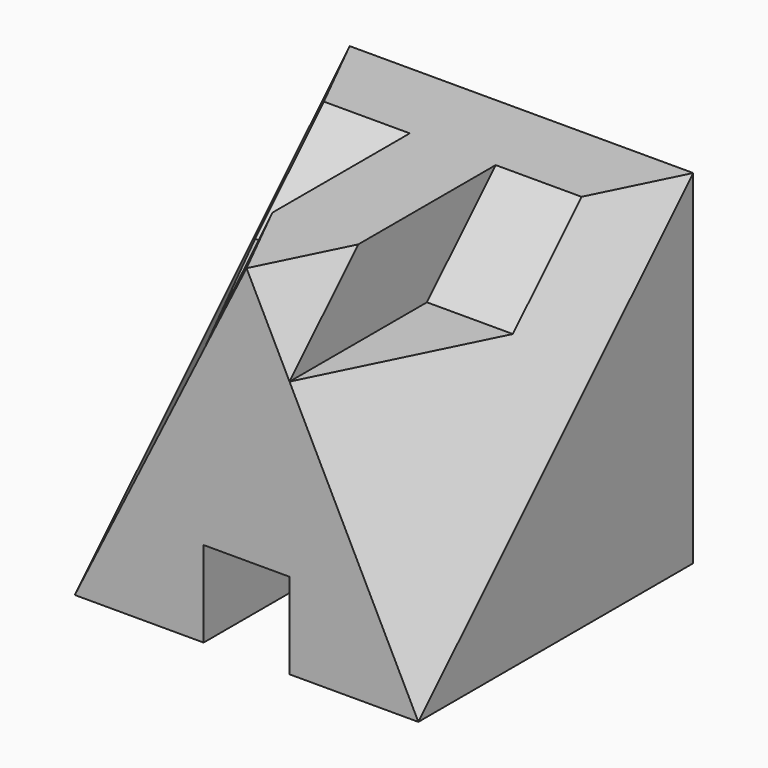
from build123d import *

# Parameters (mm, degrees)
F0_W     = 40
F0_H     = 40
F1_DEPTH = 20
F5_DEPTH = 16.3309316186
F7_DEPTH = 5
F9_DEPTH = 15


# Not quite as in the source:
# - a pattern or mirror of a feature is missing from the dataset's text; its kind, count and spacing are read off the source's solid


with BuildPart() as f1:
    # F0 (on Right) → F1 (new body, symmetric)
    with BuildSketch(Plane.YZ):
        with Locations((20, 20)):
            Rectangle(F0_W, F0_H)
    extrude(amount=F1_DEPTH, both=True)

    # F4 (on 3pt) → F5 (cut, through all)
    with BuildSketch(Plane(origin=(13.3333333333, -6.6666666667, 6.6666666667), x_dir=(-0.3651483717, -0.9128709292, -0.1825741858), z_dir=(-0.8164965809, 0.4082482905, -0.4082482905))):
        Polygon((-7.3029674334, -8.94427191), (-7.3029674334, 35.77708764), (-51.1207720338, 26.83281573), align=None)
    f5 = extrude(amount=-F5_DEPTH, mode=Mode.SUBTRACT)

    # F5_copies: F5 across plane
    add(f5.mirror(Plane(origin=(0, 0, 0), x_dir=(0, 0, -1), z_dir=(-1, 0, 0))), mode=Mode.SUBTRACT)

    # F6 (on Right) → F7 (cut, symmetric)
    with BuildSketch(Plane.YZ):
        Polygon((0, 10), (0, 0), (40, 0), align=None)
    extrude(amount=F7_DEPTH, both=True, mode=Mode.SUBTRACT)

    # F8 (on face) → F9 (cut)
    with BuildSketch(Plane.YZ.offset(20)):
        Polygon((30, 40), (10, 40), (0, 30), (20, 30), align=None)
    f9 = extrude(amount=-F9_DEPTH, mode=Mode.SUBTRACT)

    # F9_copies: F9 across plane
    add(f9.mirror(Plane(origin=(0, 0, 0), x_dir=(0, 0, -1), z_dir=(-1, 0, 0))), mode=Mode.SUBTRACT)


solid = f1.part
